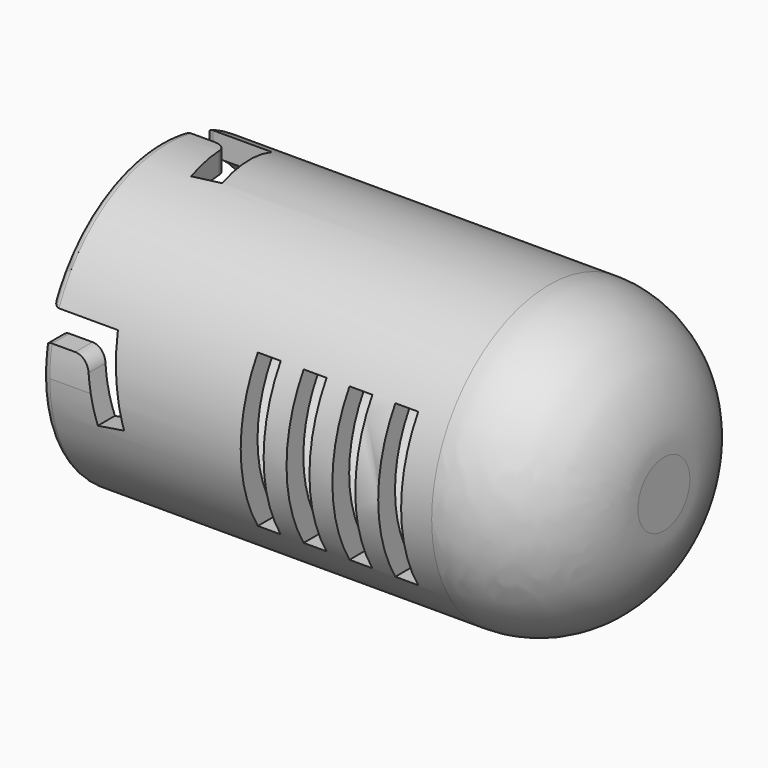
from build123d import *

# Parameters (mm, degrees)
F0_R      = 19.25
F1_DEPTH  = 1
F2_R      = 19.25
F3_DEPTH  = 65
F7_DEPTH  = 25
F10_DEPTH = 8
F14_DEPTH = 25
F16_DEPTH = 25
F17_R     = 2
F18_R     = 15
F19_W     = 3
F19_H     = 20
F20_DEPTH = 50
F21_R     = 1
F4_R      = 16.5
F22_DEPTH = 58
F23_R     = 10


with BuildPart() as f1:
    # F0 (on Right) → F1 (new body)
    with BuildSketch(Plane.YZ):
        Circle(F0_R)
    extrude(amount=F1_DEPTH)

    # F2 (on face) → F3 (join)
    with BuildSketch(Plane(origin=(0, 0, 0), x_dir=(0, -1, 0), z_dir=(-1, 0, 0))):
        Circle(F2_R)
    extrude(amount=F3_DEPTH)

    # F6 (on offset) → F7 (cut)
    with BuildSketch(Plane.XY.offset(20)):
        Polygon((-59.3079618843, 7.4748665604), (-65, 7.4748665604), (-65, 3.8748665604), (-59.3079618843, 3.8748665604), (-57.9855095289, -3.6251334396), (-54.4402016181, -3), (-56.287203212, 7.4748665604), align=None)
    extrude(amount=-F7_DEPTH, mode=Mode.SUBTRACT)

    # F9 (on offset) → F10 (cut)
    with BuildSketch(Plane.XY.offset(-20)):
        Polygon((-65, -3.8748665604), (-65, -7.4748665604), (-59.3081739576, -7.4748665604), (-56.2874152853, -7.4748665604), (-54.4404136914, 3), (-57.9857216023, 3.6251334396), (-59.3081739576, -3.8748665604), align=None)
    extrude(amount=F10_DEPTH, mode=Mode.SUBTRACT)

    # F13 (on offset) → F14 (cut)
    with BuildSketch(Plane.XZ.offset(-20)):
        Polygon((-65, -3.8748665604), (-65, -7.4748665604), (-59.3079618843, -7.4748665604), (-56.287203212, -7.4748665604), (-54.4402016181, 3), (-57.9855095289, 3.6251334396), (-59.3079618843, -3.8748665604), align=None)
    extrude(amount=F14_DEPTH, mode=Mode.SUBTRACT)

    # F15 (on offset) → F16 (cut)
    with BuildSketch(Plane.XZ.offset(20)):
        Polygon((-59.3079618843, 7.4748665604), (-65, 7.4748665604), (-65, 3.8748665604), (-59.3079618843, 3.8748665604), (-57.9855095289, -3.6251334396), (-54.4402016181, -3), (-56.287203212, 7.4748665604), align=None)
    extrude(amount=-F16_DEPTH, mode=Mode.SUBTRACT)

    # F17
    f17_edges = [f1.edges().sort_by_distance(p)[0] for p in [
        (-59.308174, -3.874867, -15.427989),
        (-59.307962, 13.165422, -3.874867),
        (-59.307962, -0.562567, -3.874867),
        (-59.307962, 3.874867, 13.165422),
        (-59.307962, 3.874867, 0),
        (-59.307962, -7.490556, 3.874867),
    ]]
    fillet(f17_edges, radius=F17_R)

    # F18
    f18_edges = [f1.edges().sort_by_distance(p)[0] for p in [
        (1, -19.25, 0),
    ]]
    fillet(f18_edges, radius=F18_R)

    # F19 (on offset) → F20 (cut)
    with BuildSketch(Plane.XZ.offset(-20)):
        with Locations((-19.5, 0)):
            Rectangle(F19_W, F19_H)
        with Locations((-25.5, 0)):
            Rectangle(F19_W, F19_H)
        with Locations((-31.5, 0)):
            Rectangle(F19_W, F19_H)
        with Locations((-37.5, 0)):
            Rectangle(F19_W, F19_H)
    extrude(amount=F20_DEPTH, mode=Mode.SUBTRACT)

    # F21
    f21_edges = [f1.edges().sort_by_distance(p)[0] for p in [
        (-65, 17.033005, 8.968793),
        (-65, 8.968793, -17.033005),
        (-65, -19.151241, 1.947424),
        (-65, -8.968793, 17.033005),
        (-65, -7.474867, -14.869736),
        (-65, -3.874867, -15.427989),
        (-65, -0.562567, -3.874867),
        (-65, 13.165422, -3.874867),
        (-65, 6.369736, -7.474867),
        (-65, 7.474867, 6.932303),
        (-65, 3.874867, 0),
        (-65, 3.874867, 13.165422),
        (-65, -7.490556, 3.874867),
        (-65, -6.932303, 7.474867),
        (-65, -16.038293, -10.645922),
    ]]
    fillet(f21_edges, radius=F21_R)

    # F4 (on face) → F22 (cut)
    with BuildSketch(Plane(origin=(-65, 0, 0), x_dir=(0, -1, 0), z_dir=(-1, 0, 0))):
        Circle(F4_R)
    extrude(amount=-F22_DEPTH, mode=Mode.SUBTRACT)

    # F23
    f23_edges = [f1.edges().sort_by_distance(p)[0] for p in [
        (-7, 16.5, 0),
    ]]
    fillet(f23_edges, radius=F23_R)


solid = f1.part
